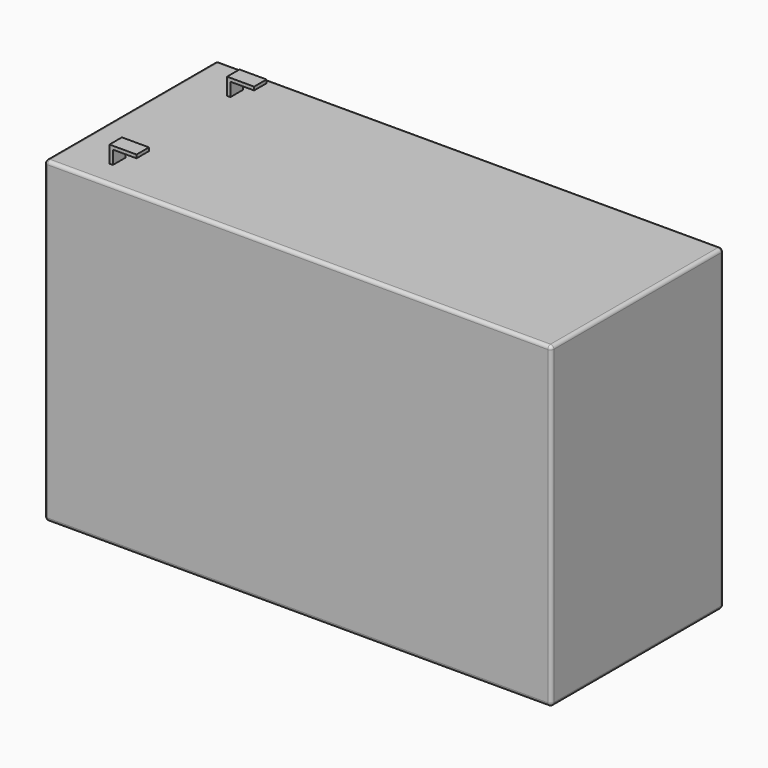
from build123d import *

# Parameters (mm, degrees)
F0_W     = 150
F0_H     = 63.8
F1_DEPTH = 94
F4_DEPTH = 2.3
F5_R     = 1


# Not quite as in the source:
# - a pattern or mirror of a feature is missing from the dataset's text; its kind, count and spacing are read off the source's solid


with BuildPart() as f1:
    # F0 (on Top) → F1 (new body)
    with BuildSketch(Plane.XY):
        Rectangle(F0_W, F0_H)
    extrude(amount=F1_DEPTH)

    # F3 (on offset) → F4 (join, symmetric)
    with BuildSketch(Plane.XZ.offset(21.75)):
        Polygon((-62, 99), (-62, 94), (-61, 94), (-61, 98), (-54, 98), (-54, 99), align=None)
    f4 = extrude(amount=F4_DEPTH, both=True)

    # F4_copies: F4 across plane
    add(f4.mirror(Plane.ZX))

    # F5
    f5_edges = [f1.edges().sort_by_distance(p)[0] for p in [
        (0, -31.9, 94),
        (75, 0, 94),
        (0, 31.9, 94),
        (-75, 0, 94),
        (-75, -31.9, 47),
        (75, -31.9, 47),
        (0, -31.9, 0),
        (75, 31.9, 47),
        (75, 0, 0),
        (-75, 31.9, 47),
        (0, 31.9, 0),
        (-75, 0, 0),
    ]]
    fillet(f5_edges, radius=F5_R)


solid = f1.part
